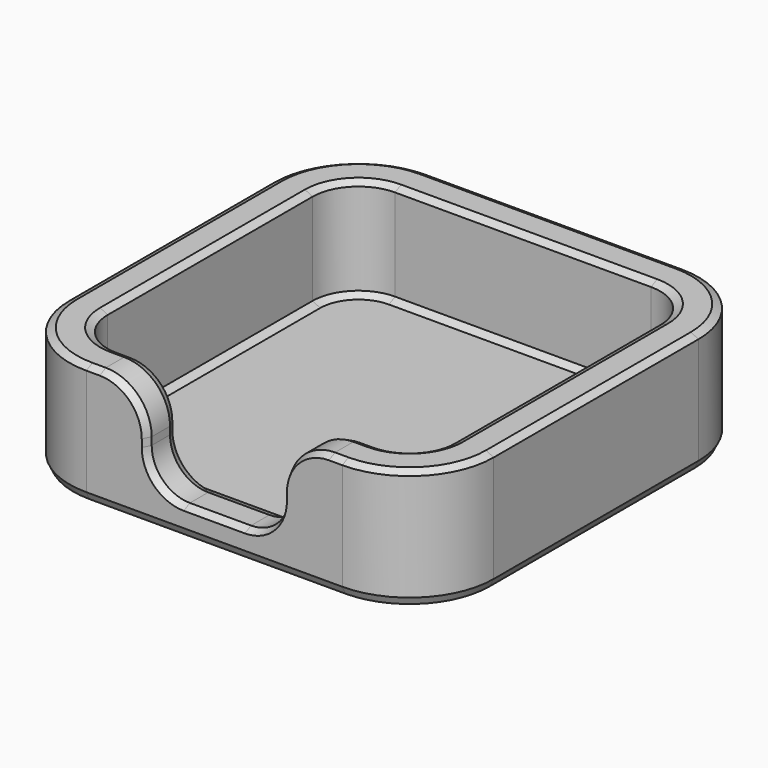
from build123d import *

# Parameters (mm, degrees)
F1_DEPTH     = 31
F3_DEPTH     = 26
F5_DEPTH     = 10
F6_T1_DEPTH  = 67
F6_T3_DEPTH  = 67
F6_T6_ANGLE  = 90
F6_T8_ANGLE  = 90
F6_T10_ANGLE = 90
F6_T12_ANGLE = 90
F6_T13_DEPTH = 67
F6_T15_DEPTH = 67
F6_T17_DEPTH = 3.5
F6_T19_DEPTH = 3.5
F6_T21_DEPTH = 2
F6_T23_DEPTH = 16
F6_T26_ANGLE = 90
F6_T28_ANGLE = 90
F6_T30_ANGLE = 90
F6_T32_ANGLE = 90
F6_T34_ANGLE = 90
F6_T36_ANGLE = 90
F6_T38_ANGLE = 90
F6_T40_ANGLE = 90
F6_T42_ANGLE = 90
F6_T44_ANGLE = 90
F6_T46_ANGLE = 90
F6_T48_ANGLE = 90
F6_T50_ANGLE = 90
F6_T52_ANGLE = 90
F6_T54_ANGLE = 90
F6_T56_ANGLE = 90
F6_T58_ANGLE = 90
F6_T60_ANGLE = 90
F6_T62_ANGLE = 90
F6_T64_ANGLE = 90


# Not quite as in the source:
# - a fillet or chamfer that OpenCascade refuses, or shapes differently, is made with other operations: its cross-section is extruded or revolved along the edge and cut away or added


with BuildPart() as f1:
    # F0 (on Top) → F1 (new body)
    with BuildSketch(Plane.XY):
        with BuildLine():
            Line((55.5, -33.5), (55.5, 33.5))
            ThreePointArc((55.5, 33.5), (49.0563491861, 49.0563491861), (33.5, 55.5))
            Line((33.5, 55.5), (-33.5, 55.5))
            ThreePointArc((-33.5, 55.5), (-49.0563491861, 49.0563491861), (-55.5, 33.5))
            Line((-55.5, 33.5), (-55.5, -33.5))
            ThreePointArc((-55.5, -33.5), (-49.0563491861, -49.0563491861), (-33.5, -55.5))
            Line((-33.5, -55.5), (33.5, -55.5))
            ThreePointArc((33.5, -55.5), (49.0563491861, -49.0563491861), (55.5, -33.5))
        make_face()
    extrude(amount=F1_DEPTH)

    # F2 (on face) → F3 (cut, through all)
    with BuildSketch(Plane.XY.offset(31)):
        with BuildLine():
            Line((33.5, 45.5), (-33.5, 45.5))
            ThreePointArc((-33.5, 45.5), (-41.9852813742, 41.9852813742), (-45.5, 33.5))
            Line((-45.5, 33.5), (-45.5, -33.5))
            ThreePointArc((-45.5, -33.5), (-41.9852813742, -41.9852813742), (-33.5, -45.5))
            Line((-33.5, -45.5), (33.5, -45.5))
            ThreePointArc((33.5, -45.5), (41.9852813742, -41.9852813742), (45.5, -33.5))
            Line((45.5, -33.5), (45.5, 33.5))
            ThreePointArc((45.5, 33.5), (41.9852813742, 41.9852813742), (33.5, 45.5))
        make_face()
    extrude(amount=-F3_DEPTH, mode=Mode.SUBTRACT)

    # F4 (on face) → F5 (cut, through all)
    with BuildSketch(Plane.XZ.offset(55.5)):
        with BuildLine():
            ThreePointArc((-30, 31), (-21.5147186258, 27.4852813742), (-18, 19))
            Line((-18, 19), (-18, 17))
            ThreePointArc((-18, 17), (-15.0710678119, 9.9289321881), (-8, 7))
            Line((-8, 7), (8, 7))
            ThreePointArc((8, 7), (15.0710678119, 9.9289321881), (18, 17))
            Line((18, 17), (18, 19))
            ThreePointArc((18, 19), (21.5147186258, 27.4852813742), (30, 31))
            Line((30, 31), (-30, 31))
        make_face()
    extrude(amount=-F5_DEPTH, mode=Mode.SUBTRACT)

    # F6: chamfer of 2 x 1 on 48 edges, made by hand

    # F6_s2 → F6_t1 (join)
    with BuildSketch(Plane.XZ.offset(-33.5)):
        Polygon((-45.5, 6), (-43.5, 5), (-45.5, 5), align=None)
        Polygon((45.5, 6), (43.5, 5), (45.5, 5), align=None)
    extrude(amount=F6_T1_DEPTH)

    # F6_s4 → F6_t3 (join)
    with BuildSketch(Plane.YZ.offset(-33.5)):
        Polygon((-45.5, 6), (-43.5, 5), (-45.5, 5), align=None)
        Polygon((45.5, 6), (43.5, 5), (45.5, 5), align=None)
    extrude(amount=F6_T3_DEPTH)

    # F6_s5 → F6_t6 (revolve)
    with BuildSketch(Plane.YZ.offset(33.5)):
        Polygon((-45.5, 6), (-43.5, 5), (-45.5, 5), align=None)
    revolve(axis=Axis((33.5, -33.5, 5), (0, 0, 1)), revolution_arc=F6_T6_ANGLE)

    # F6_s7 → F6_t8 (revolve)
    with BuildSketch(Plane.XZ.offset(-33.5)):
        Polygon((45.5, 6), (43.5, 5), (45.5, 5), align=None)
    revolve(axis=Axis((33.5, 33.5, 5), (0, 0, 1)), revolution_arc=F6_T8_ANGLE)

    # F6_s9 → F6_t10 (revolve)
    with BuildSketch(Plane.YZ.offset(-33.5)):
        Polygon((45.5, 6), (43.5, 5), (45.5, 5), align=None)
    revolve(axis=Axis((-33.5, 33.5, 5), (0, 0, 1)), revolution_arc=F6_T10_ANGLE)

    # F6_s11 → F6_t12 (revolve)
    with BuildSketch(Plane.XZ.offset(33.5)):
        Polygon((-45.5, 6), (-43.5, 5), (-45.5, 5), align=None)
    revolve(axis=Axis((-33.5, -33.5, 5), (0, 0, 1)), revolution_arc=F6_T12_ANGLE)

    # F6_s14 → F6_t13 (cut)
    with BuildSketch(Plane.YZ.offset(-33.5)):
        Polygon((47.5, 31), (45.5, 30), (45.5, 31), align=None)
        Polygon((53.5, 31), (55.5, 30), (55.5, 31), align=None)
        Polygon((-54.5, 0), (-55.5, 2), (-55.5, 0), align=None)
        Polygon((54.5, 0), (55.5, 2), (55.5, 0), align=None)
    extrude(amount=F6_T13_DEPTH, mode=Mode.SUBTRACT)

    # F6_s16 → F6_t15 (cut)
    with BuildSketch(Plane.XZ.offset(-33.5)):
        Polygon((55.5, 2), (54.5, 0), (55.5, 0), align=None)
        Polygon((55.5, 30), (53.5, 31), (55.5, 31), align=None)
        Polygon((-54.5, 0), (-55.5, 2), (-55.5, 0), align=None)
        Polygon((47.5, 31), (45.5, 30), (45.5, 31), align=None)
        Polygon((-47.5, 31), (-45.5, 30), (-45.5, 31), align=None)
        Polygon((-53.5, 31), (-55.5, 30), (-55.5, 31), align=None)
    extrude(amount=F6_T15_DEPTH, mode=Mode.SUBTRACT)

    # F6_s18 → F6_t17 (cut)
    with BuildSketch(Plane.YZ.offset(30)):
        Polygon((-53.5, 31), (-55.5, 30), (-55.5, 31), align=None)
        Polygon((-47.5, 31), (-45.5, 30), (-45.5, 31), align=None)
    extrude(amount=F6_T17_DEPTH, mode=Mode.SUBTRACT)

    # F6_s20 → F6_t19 (cut)
    with BuildSketch(Plane.YZ.offset(-33.5)):
        Polygon((-47.5, 31), (-45.5, 30), (-45.5, 31), align=None)
        Polygon((-53.5, 31), (-55.5, 30), (-55.5, 31), align=None)
    extrude(amount=F6_T19_DEPTH, mode=Mode.SUBTRACT)

    # F6_s22 → F6_t21 (cut)
    with BuildSketch(Plane.XY.offset(17)):
        Polygon((19, -55.5), (18, -53.5), (18, -55.5), align=None)
        Polygon((-19, -55.5), (-18, -53.5), (-18, -55.5), align=None)
        Polygon((-19, -45.5), (-18, -47.5), (-18, -45.5), align=None)
        Polygon((19, -45.5), (18, -47.5), (18, -45.5), align=None)
    extrude(amount=F6_T21_DEPTH, mode=Mode.SUBTRACT)

    # F6_s24 → F6_t23 (cut)
    with BuildSketch(Plane.YZ.offset(-8)):
        Polygon((-55.5, 6), (-53.5, 7), (-55.5, 7), align=None)
        Polygon((-45.5, 6), (-47.5, 7), (-45.5, 7), align=None)
    extrude(amount=F6_T23_DEPTH, mode=Mode.SUBTRACT)

    # F6_s25 → F6_t26 (revolve, cut)
    with BuildSketch(Plane.YZ.offset(33.5)):
        Polygon((-55.5, 2), (-54.5, 0), (-55.5, 0), align=None)
    revolve(axis=Axis((33.5, -33.5, 0), (0, 0, 1)), revolution_arc=F6_T26_ANGLE, mode=Mode.SUBTRACT)

    # F6_s27 → F6_t28 (revolve, cut)
    with BuildSketch(Plane.YZ.offset(33.5)):
        Polygon((-55.5, 30), (-53.5, 31), (-55.5, 31), align=None)
    revolve(axis=Axis((33.5, -33.5, 31), (0, 0, 1)), revolution_arc=F6_T28_ANGLE, mode=Mode.SUBTRACT)

    # F6_s29 → F6_t30 (revolve, cut)
    with BuildSketch(Plane.XZ.offset(-33.5)):
        Polygon((55.5, 2), (54.5, 0), (55.5, 0), align=None)
    revolve(axis=Axis((33.5, 33.5, 0), (0, 0, 1)), revolution_arc=F6_T30_ANGLE, mode=Mode.SUBTRACT)

    # F6_s31 → F6_t32 (revolve, cut)
    with BuildSketch(Plane.XZ.offset(-33.5)):
        Polygon((55.5, 30), (53.5, 31), (55.5, 31), align=None)
    revolve(axis=Axis((33.5, 33.5, 31), (0, 0, 1)), revolution_arc=F6_T32_ANGLE, mode=Mode.SUBTRACT)

    # F6_s33 → F6_t34 (revolve, cut)
    with BuildSketch(Plane.YZ.offset(-33.5)):
        Polygon((54.5, 0), (55.5, 2), (55.5, 0), align=None)
    revolve(axis=Axis((-33.5, 33.5, 0), (0, 0, 1)), revolution_arc=F6_T34_ANGLE, mode=Mode.SUBTRACT)

    # F6_s35 → F6_t36 (revolve, cut)
    with BuildSketch(Plane.XZ.offset(33.5)):
        Polygon((-54.5, 0), (-55.5, 2), (-55.5, 0), align=None)
    revolve(axis=Axis((-33.5, -33.5, 0), (0, 0, 1)), revolution_arc=F6_T36_ANGLE, mode=Mode.SUBTRACT)

    # F6_s37 → F6_t38 (revolve, cut)
    with BuildSketch(Plane.YZ.offset(33.5)):
        Polygon((-47.5, 31), (-45.5, 30), (-45.5, 31), align=None)
    revolve(axis=Axis((33.5, -33.5, 31), (0, 0, 1)), revolution_arc=F6_T38_ANGLE, mode=Mode.SUBTRACT)

    # F6_s39 → F6_t40 (revolve, cut)
    with BuildSketch(Plane.XZ.offset(-33.5)):
        Polygon((47.5, 31), (45.5, 30), (45.5, 31), align=None)
    revolve(axis=Axis((33.5, 33.5, 31), (0, 0, 1)), revolution_arc=F6_T40_ANGLE, mode=Mode.SUBTRACT)

    # F6_s41 → F6_t42 (revolve, cut)
    with BuildSketch(Plane.YZ.offset(-33.5)):
        Polygon((47.5, 31), (45.5, 30), (45.5, 31), align=None)
    revolve(axis=Axis((-33.5, 33.5, 31), (0, 0, 1)), revolution_arc=F6_T42_ANGLE, mode=Mode.SUBTRACT)

    # F6_s43 → F6_t44 (revolve, cut)
    with BuildSketch(Plane.XZ.offset(33.5)):
        Polygon((-47.5, 31), (-45.5, 30), (-45.5, 31), align=None)
    revolve(axis=Axis((-33.5, -33.5, 31), (0, 0, 1)), revolution_arc=F6_T44_ANGLE, mode=Mode.SUBTRACT)

    # F6_s45 → F6_t46 (revolve, cut)
    with BuildSketch(Plane.XZ.offset(33.5)):
        Polygon((-53.5, 31), (-55.5, 30), (-55.5, 31), align=None)
    revolve(axis=Axis((-33.5, -33.5, 31), (0, 0, 1)), revolution_arc=F6_T46_ANGLE, mode=Mode.SUBTRACT)

    # F6_s47 → F6_t48 (revolve, cut)
    with BuildSketch(Plane.YZ.offset(-33.5)):
        Polygon((53.5, 31), (55.5, 30), (55.5, 31), align=None)
    revolve(axis=Axis((-33.5, 33.5, 31), (0, 0, 1)), revolution_arc=F6_T48_ANGLE, mode=Mode.SUBTRACT)

    # F6_s49 → F6_t50 (revolve, cut)
    with BuildSketch(Plane.XY.offset(19)):
        Polygon((19, -55.5), (18, -53.5), (18, -55.5), align=None)
    revolve(axis=Axis((30, -55.5, 19), (0, 1, 0)), revolution_arc=F6_T50_ANGLE, mode=Mode.SUBTRACT)

    # F6_s51 → F6_t52 (revolve, cut)
    with BuildSketch(Plane.YZ.offset(8)):
        Polygon((-55.5, 6), (-53.5, 7), (-55.5, 7), align=None)
    revolve(axis=Axis((8, -55.5, 17), (0, -1, 0)), revolution_arc=F6_T52_ANGLE, mode=Mode.SUBTRACT)

    # F6_s53 → F6_t54 (revolve, cut)
    with BuildSketch(Plane.XY.offset(17)):
        Polygon((-19, -55.5), (-18, -53.5), (-18, -55.5), align=None)
    revolve(axis=Axis((-8, -55.5, 17), (0, -1, 0)), revolution_arc=F6_T54_ANGLE, mode=Mode.SUBTRACT)

    # F6_s55 → F6_t56 (revolve, cut)
    with BuildSketch(Plane.YZ.offset(-30)):
        Polygon((-55.5, 30), (-53.5, 31), (-55.5, 31), align=None)
    revolve(axis=Axis((-30, -55.5, 19), (0, 1, 0)), revolution_arc=F6_T56_ANGLE, mode=Mode.SUBTRACT)

    # F6_s57 → F6_t58 (revolve, cut)
    with BuildSketch(Plane.XY.offset(19)):
        Polygon((18, -47.5), (19, -45.5), (18, -45.5), align=None)
    revolve(axis=Axis((30, -45.5, 19), (0, 1, 0)), revolution_arc=F6_T58_ANGLE, mode=Mode.SUBTRACT)

    # F6_s59 → F6_t60 (revolve, cut)
    with BuildSketch(Plane.YZ.offset(-30)):
        Polygon((-45.5, 30), (-47.5, 31), (-45.5, 31), align=None)
    revolve(axis=Axis((-30, -45.5, 19), (0, 1, 0)), revolution_arc=F6_T60_ANGLE, mode=Mode.SUBTRACT)

    # F6_s61 → F6_t62 (revolve, cut)
    with BuildSketch(Plane.XY.offset(17)):
        Polygon((-19, -45.5), (-18, -47.5), (-18, -45.5), align=None)
    revolve(axis=Axis((-8, -45.5, 17), (0, -1, 0)), revolution_arc=F6_T62_ANGLE, mode=Mode.SUBTRACT)

    # F6_s63 → F6_t64 (revolve, cut)
    with BuildSketch(Plane.YZ.offset(8)):
        Polygon((-45.5, 6), (-47.5, 7), (-45.5, 7), align=None)
    revolve(axis=Axis((8, -45.5, 17), (0, -1, 0)), revolution_arc=F6_T64_ANGLE, mode=Mode.SUBTRACT)


solid = f1.part
